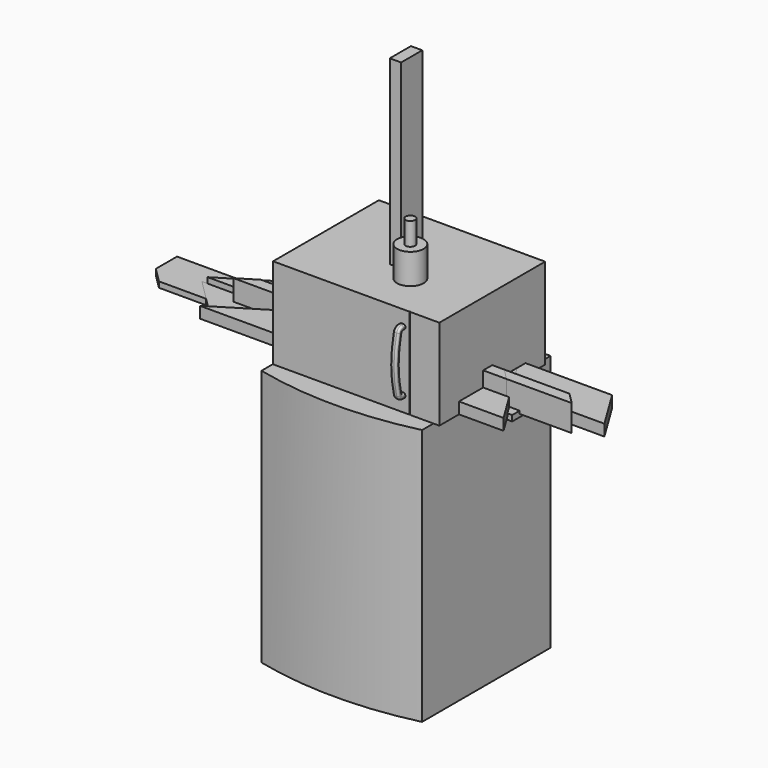
from build123d import *

# Parameters (mm, degrees)
F0_W      = 539.75
F0_H      = 539.75
F0_R      = 63.5
F0_R_2    = 44.45
F1_DEPTH  = 863.6
F2_DEPTH  = 406.4
F3_DEPTH  = 9.525
F6_R      = 15.875
F7_DEPTH  = 76.2
F8_W      = 558.8
F8_H      = 444.5
F9_DEPTH  = 304.8
F14_W     = 3.175
F14_H     = 304.8
F15_DEPTH = 1.5875
F16_W     = 139.7
F16_H     = 19.05
F17_DEPTH = 412.75
F19_DEPTH = 19.05
F21_DEPTH = 19.05
F22_W     = 38.1
F22_H     = 88.9
F23_DEPTH = 914.4
F25_DEPTH = 38.1
F27_DEPTH = 88.9
F29_DEPTH = 88.9
F30_SIZE2 = 23.807512
F30_SIZE  = 38.09999
F31_SIZE2 = 62.173539
F31_SIZE  = 38.09999
F33_DEPTH = 38.1
F35_DEPTH = 38.1
F36_R     = 22.225
F37_DEPTH = 38.1


# Not quite as in the source:
# - a fillet or chamfer is up to 0.001 mm smaller than in the source, because OpenCascade refuses the exact size


with BuildPart() as f1:
    # F0 (on Top) → F1 (new body)
    with BuildSketch(Plane.XY):
        Rectangle(F0_W, F0_H)
        with Locations((73.025, -73.025)):
            Circle(F0_R, mode=Mode.SUBTRACT)
        with BuildLine():
            ThreePointArc((-269.875, -269.875), (0, -301.625), (269.875, -269.875))
            Line((269.875, -269.875), (-269.875, -269.875))
        make_face()
        with Locations((73.025, -73.025)):
            Circle(F0_R)
        with Locations((73.025, -73.025)):
            Circle(F0_R_2, mode=Mode.SUBTRACT)
        with Locations((73.025, -73.025)):
            Circle(F0_R_2)
    extrude(amount=-F1_DEPTH)

    # F0 (on Top) → F2 (join)
    with BuildSketch(Plane.XY):
        with Locations((73.025, -73.025)):
            Circle(F0_R_2)
    extrude(amount=F2_DEPTH)

    # F0 (on Top) → F3 (join)
    with BuildSketch(Plane.XY):
        with Locations((73.025, -73.025)):
            Circle(F0_R)
        with Locations((73.025, -73.025)):
            Circle(F0_R_2, mode=Mode.SUBTRACT)
    extrude(amount=F3_DEPTH)

    # F6 (on face) → F7 (join)
    with BuildSketch(Plane.XY.offset(406.4)):
        with Locations((73.025, -73.025)):
            Circle(F6_R)
    extrude(amount=F7_DEPTH)


with BuildPart() as f9:
    # F8 (on Top) → F9 (new body)
    with BuildSketch(Plane.XY):
        with Locations((10.3976642355, 0)):
            Rectangle(F8_W, F8_H)
    extrude(amount=F9_DEPTH)

    # F13: sweep along a path in F12
    with BuildLine(Plane.YZ.offset(161.925)) as f13_path:
        Line((-222.25, 254), (-230.4096808985, 254))
        ThreePointArc((-230.4096808985, 254), (-238.2313792766, 251.3055501839), (-242.7341526537, 244.3655172414))
        ThreePointArc((-242.7341526537, 244.3655172414), (-254, 152.4), (-242.7341526537, 60.4344827586))
        ThreePointArc((-242.7341526537, 60.4344827586), (-238.2313792766, 53.4944498161), (-230.4096808985, 50.8))
        Line((-230.4096808985, 50.8), (-222.25, 50.8))
    # F10 (on face) → F13 (sweep)
    with BuildSketch(Plane.XZ.offset(222.25)):
        with BuildLine():
            Line((162.7976642355, 246.0625), (169.1476642355, 246.0625))
            ThreePointArc((169.1476642355, 246.0625), (173.637792296, 247.9223719395), (175.4976642355, 252.4125))
            Line((175.4976642355, 252.4125), (175.4976642355, 255.5875))
            ThreePointArc((175.4976642355, 255.5875), (173.637792296, 260.0776280605), (169.1476642355, 261.9375))
            Line((169.1476642355, 261.9375), (162.7976642355, 261.9375))
            ThreePointArc((162.7976642355, 261.9375), (158.3075361749, 260.0776280605), (156.4476642355, 255.5875))
            Line((156.4476642355, 255.5875), (156.4476642355, 252.4125))
            ThreePointArc((156.4476642355, 252.4125), (158.3075361749, 247.9223719395), (162.7976642355, 246.0625))
        make_face()
    sweep(path=f13_path.line)

    # F14 (on face) → F15 (cut)
    with BuildSketch(Plane.XZ.offset(222.25)):
        with Locations((191.0551642355, 152.4)):
            Rectangle(F14_W, F14_H)
    extrude(amount=-F15_DEPTH, mode=Mode.SUBTRACT)


with BuildPart() as f17:
    # F16 (on Right) → F17 (new body, symmetric)
    with BuildSketch(Plane.YZ):
        Rectangle(F16_W, F16_H)
    extrude(amount=F17_DEPTH, both=True)


with BuildPart() as f19:
    # F18 (on Top) → F19 (new body)
    with BuildSketch(Plane.XY):
        Polygon((-825.5, -19.05), (-774.7, -69.85), (0, -69.85), (0, 69.85), (-825.5, 69.85), align=None)
    extrude(amount=F19_DEPTH)


with BuildPart() as f21:
    # F20 (on Top) → F21 (new body)
    with BuildSketch(Plane.XY):
        Polygon((0, -139.7), (0, 0), (-685.8, 0), (-546.1, -139.7), align=None)
    extrude(amount=F21_DEPTH)


with BuildPart() as f23:
    # F22 (on Top) → F23 (new body, symmetric)
    with BuildSketch(Plane.XY):
        Rectangle(F22_W, F22_H)
    extrude(amount=F23_DEPTH, both=True)


with BuildPart() as f25:
    # F24 (on Top) → F25 (new body)
    with BuildSketch(Plane.XY):
        Polygon((-666.75, 0), (666.75, 0), (581.0462384661, 139.7), (-439.5653237969, 139.7), align=None)
    extrude(amount=F25_DEPTH)


with BuildPart() as f27:
    # F26 (on Top) → F27 (new body)
    with BuildSketch(Plane.XY):
        Polygon((549.275, 0), (-549.275, 0), (-549.275, -38.1), (587.375, -38.1), align=None)
    extrude(amount=F27_DEPTH)

    # F31 (size 38.1 and 62.1735492796 in the source; OpenCascade refuses exactly that, so slightly less here)
    f31_edges = [f27.edges().sort_by_distance(p)[0] for p in [
        (-549.275, 0, 44.45),
    ]]
    f31_side = f27.faces().sort_by_distance((-549.275, -19.05, 44.45))[0]
    chamfer(f31_edges, length=F31_SIZE, length2=F31_SIZE2, reference=f31_side)


with BuildPart() as f29:
    # F28 (on Top) → F29 (new body)
    with BuildSketch(Plane.XY):
        Polygon((330.2, 0), (-330.2, 0), (-330.2, -38.1), (368.3, -38.1), align=None)
    extrude(amount=F29_DEPTH)

    # F30 (size 38.1 and 23.8075223077 in the source; OpenCascade refuses exactly that, so slightly less here)
    f30_edges = [f29.edges().sort_by_distance(p)[0] for p in [
        (-330.2, 0, 44.45),
    ]]
    f30_side = f29.faces().sort_by_distance((-330.2, -19.05, 44.45))[0]
    chamfer(f30_edges, length=F30_SIZE, length2=F30_SIZE2, reference=f30_side)


with BuildPart() as f33:
    # F32 (on Top) → F33 (new body)
    with BuildSketch(Plane.XY):
        Polygon((-581.0518573346, -139.7), (439.5709426654, -139.7), (353.8671811315, 0), (-353.8671811315, 0), align=None)
    extrude(amount=F33_DEPTH)


with BuildPart() as f35:
    # F34 (on Top) → F35 (new body)
    with BuildSketch(Plane.XY):
        Polygon((-353.8728, 0), (353.8728, 0), (268.1690384661, 139.7), (-126.6881237969, 139.7), align=None)
    extrude(amount=F35_DEPTH)


with BuildPart() as f37:
    # F36 (on Top) → F37 (new body)
    with BuildSketch(Plane.XY):
        Polygon((-197.4342, 0), (197.4342, 0), (111.7304384661, 139.7), (29.7504762031, 139.7), align=None)
        with Locations((34.2739268669, 71.6638964194)):
            Circle(F36_R, mode=Mode.SUBTRACT)
    extrude(amount=F37_DEPTH)


solid = Compound([f1.part, f9.part, f17.part, f19.part, f21.part, f23.part, f25.part, f27.part, f29.part, f33.part, f35.part, f37.part])
